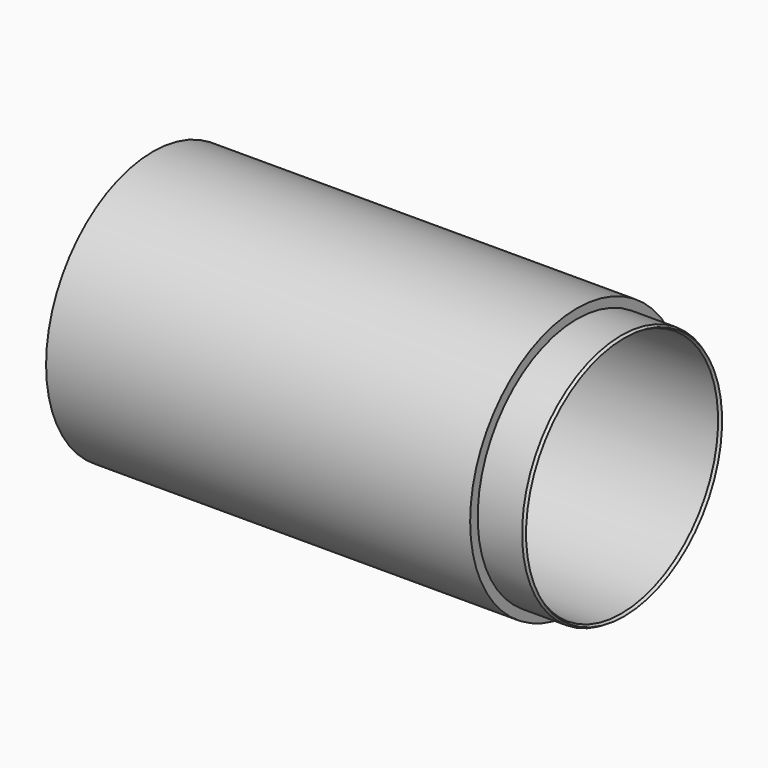
from build123d import *

# Parameters (mm, degrees)
F2_SIZE2 = 0.21996
F2_SIZE  = 0.12699


# Not quite as in the source:
# - a fillet or chamfer is up to 0.001 mm smaller than in the source, because OpenCascade refuses the exact size


with BuildPart() as f1:
    # F0 (on Front) → F1 (revolve)
    with BuildSketch(Plane.XZ):
        Polygon((-38.1, 9.779), (0, 9.779), (0, 10.033), (-3.81, 10.033), (-3.81, 10.795), (-38.1, 10.795), align=None)
    revolve(axis=Axis((-19.05, 0, 0), (-1, 0, 0)))

    # F2 (size 0.127 and 0.2199704526 in the source; OpenCascade refuses exactly that, so slightly less here)
    f2_edges = [f1.edges().sort_by_distance(p)[0] for p in [
        (0, 0, -10.033),
        (0, 0, -9.779),
    ]]
    f2_side = f1.faces().sort_by_distance((0, 0, -9.807378))[0]
    chamfer(f2_edges, length=F2_SIZE, length2=F2_SIZE2, reference=f2_side)


solid = f1.part
